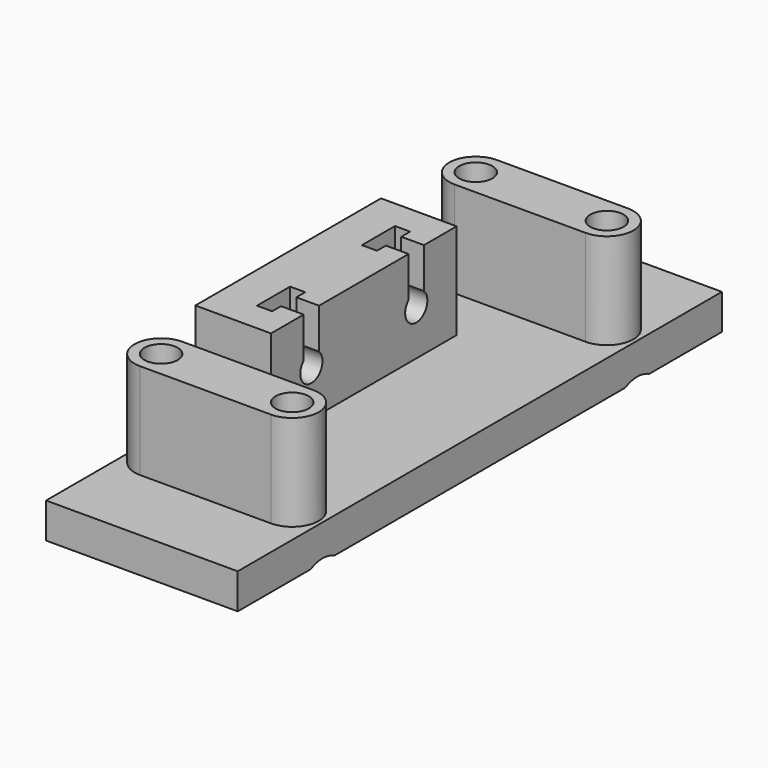
from build123d import *

# Parameters (mm, degrees)
F0_W           = 15
F0_H           = 46
F0_R           = 2.5
F1_DEPTH       = 7
F2_DEPTH       = 19
F4_D           = 5.5
F4_CBORE_D     = 9.75
F4_CBORE_DEPTH = 5
F5_W           = 3
F5_H           = 8.2
F6_DEPTH       = 20
F8_D           = 6.6
F8_DEPTH       = 40
F8_CSINK_D     = 13.44
F8_CSINK_ANGLE = 90
F8_TIP         = 1.9828400428
F9_W           = 4.5
F9_H           = 3.8
F10_DEPTH      = 10


# Not quite as in the source:
# - a feature names something its author has since deleted; it is built from what else it names


with BuildPart() as f1:
    # F0 (on Top) → F1 (new body)
    with BuildSketch(Plane.XY):
        Polygon((-80, -60), (-80, 60), (-118, 60), (-118, 23), (-103, 23), (-103, -23), (-118, -23), (-118, -60), align=None)
        with BuildLine():
            Line((-86, -44.25), (-112, -44.25))
            ThreePointArc((-112, -44.25), (-117.25, -39), (-112, -33.75))
            Line((-112, -33.75), (-86, -33.75))
            ThreePointArc((-86, -33.75), (-80.75, -39), (-86, -44.25))
        make_face(mode=Mode.SUBTRACT)
        with BuildLine():
            Line((-86, 33.75), (-112, 33.75))
            ThreePointArc((-112, 33.75), (-117.25, 39), (-112, 44.25))
            Line((-112, 44.25), (-86, 44.25))
            ThreePointArc((-86, 44.25), (-80.75, 39), (-86, 33.75))
        make_face(mode=Mode.SUBTRACT)
        with Locations((-110.5, 0)):
            Rectangle(F0_W, F0_H)
        with BuildLine():
            ThreePointArc((-112, 44.25), (-117.25, 39), (-112, 33.75))
            Line((-112, 33.75), (-86, 33.75))
            ThreePointArc((-86, 33.75), (-80.75, 39), (-86, 44.25))
            Line((-86, 44.25), (-112, 44.25))
        make_face()
        with Locations((-112, 39)):
            Circle(F0_R, mode=Mode.SUBTRACT)
        with Locations((-86, 39)):
            Circle(F0_R, mode=Mode.SUBTRACT)
        with BuildLine():
            ThreePointArc((-112, -33.75), (-117.25, -39), (-112, -44.25))
            Line((-112, -44.25), (-86, -44.25))
            ThreePointArc((-86, -44.25), (-80.75, -39), (-86, -33.75))
            Line((-86, -33.75), (-112, -33.75))
        make_face()
        with Locations((-112, -39)):
            Circle(F0_R, mode=Mode.SUBTRACT)
        with BuildLine():
            ThreePointArc((-83.5, -39), (-86, -41.5), (-88.5, -39))
            ThreePointArc((-88.5, -39), (-86, -36.5), (-83.5, -39))
        make_face(mode=Mode.SUBTRACT)
        with Locations((-112, 39)):
            Circle(F0_R)
        with Locations((-86, 39)):
            Circle(F0_R)
        with Locations((-112, -39)):
            Circle(F0_R)
        with BuildLine():
            ThreePointArc((-83.5, -39), (-86, -36.5), (-88.5, -39))
            ThreePointArc((-88.5, -39), (-86, -41.5), (-83.5, -39))
        make_face()
    extrude(amount=-F1_DEPTH)

    # F0 (on Top) → F2 (join)
    with BuildSketch(Plane.XY):
        with BuildLine():
            ThreePointArc((-112, 44.25), (-117.25, 39), (-112, 33.75))
            Line((-112, 33.75), (-86, 33.75))
            ThreePointArc((-86, 33.75), (-80.75, 39), (-86, 44.25))
            Line((-86, 44.25), (-112, 44.25))
        make_face()
        with Locations((-112, 39)):
            Circle(F0_R, mode=Mode.SUBTRACT)
        with Locations((-86, 39)):
            Circle(F0_R, mode=Mode.SUBTRACT)
        with BuildLine():
            ThreePointArc((-112, -33.75), (-117.25, -39), (-112, -44.25))
            Line((-112, -44.25), (-86, -44.25))
            ThreePointArc((-86, -44.25), (-80.75, -39), (-86, -33.75))
            Line((-86, -33.75), (-112, -33.75))
        make_face()
        with Locations((-112, -39)):
            Circle(F0_R, mode=Mode.SUBTRACT)
        with BuildLine():
            ThreePointArc((-83.5, -39), (-86, -41.5), (-88.5, -39))
            ThreePointArc((-88.5, -39), (-86, -36.5), (-83.5, -39))
        make_face(mode=Mode.SUBTRACT)
        with Locations((-110.5, 0)):
            Rectangle(F0_W, F0_H)
        with Locations((-112, 39)):
            Circle(F0_R)
        with Locations((-86, 39)):
            Circle(F0_R)
        with BuildLine():
            ThreePointArc((-83.5, -39), (-86, -36.5), (-88.5, -39))
            ThreePointArc((-88.5, -39), (-86, -41.5), (-83.5, -39))
        make_face()
        with Locations((-112, -39)):
            Circle(F0_R)
    extrude(amount=F2_DEPTH)

    # F4 (through all)
    with Locations(Plane(origin=(-118, 0, 0), x_dir=(0, -1, 0), z_dir=(-1, 0, 0))):
        with Locations((-13, 9), (13, 9)):
            CounterBoreHole(F4_D / 2, F4_CBORE_D / 2, F4_CBORE_DEPTH)

    # F5 (on face) → F6 (cut)
    with BuildSketch(Plane.XY.offset(19)):
        with Locations((-109, 13)):
            Rectangle(F5_W, F5_H)
        with Locations((-109, -13)):
            Rectangle(F5_W, F5_H)
    extrude(amount=-F6_DEPTH, mode=Mode.SUBTRACT)

    # F8
    with Locations(Plane(origin=(0, 0, -7), x_dir=(1, 0, 0), z_dir=(0, 0, -1))):
        with Locations((-86, -39), (-112, -39), (-112, 39), (-86, 39)):
            CounterSinkHole(F8_D / 2, F8_CSINK_D / 2, depth=F8_DEPTH, counter_sink_angle=F8_CSINK_ANGLE)
            with Locations((0, 0, -(F8_DEPTH + F8_TIP / 2))):  # 118° drill point
                Cone(0, F8_D / 2, F8_TIP, mode=Mode.SUBTRACT)

    # F9 (on face) → F10 (cut)
    with BuildSketch(Plane.XY.offset(19)):
        with Locations((-105.25, 13)):
            Rectangle(F9_W, F9_H)
        with Locations((-105.25, -13)):
            Rectangle(F9_W, F9_H)
    extrude(amount=-F10_DEPTH, mode=Mode.SUBTRACT)


solid = f1.part
